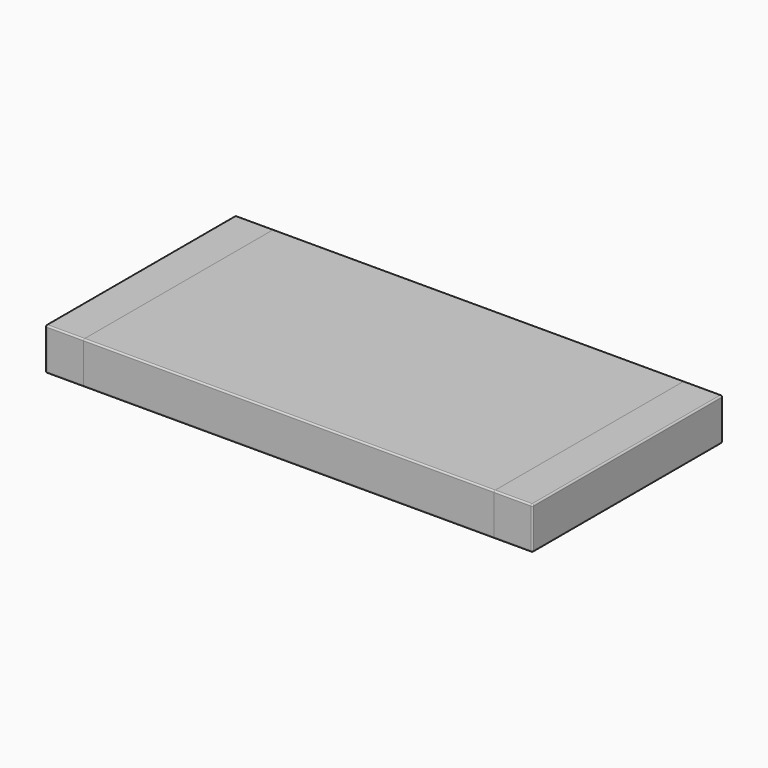
from build123d import *

# Parameters (mm, degrees)
F2_W     = 5.35
F2_H     = 3.1
F3_DEPTH = 0.53
F2_W_2   = 0.5
F4_DEPTH = 0.55
F5_DEPTH = 0.55
F6_DEPTH = 0.02
F7_R     = 0.01999
F7_2_R   = 0.01999
F7_3_R   = 0.01999
F7_4_R   = 0.01999


# Not quite as in the source:
# - a fillet or chamfer is up to 0.001 mm smaller than in the source, because OpenCascade refuses the exact size


with BuildPart() as f3:
    # F2 (on Top) → F3 (new body)
    with BuildSketch(Plane.XY):
        Rectangle(F2_W, F2_H)
    extrude(amount=F3_DEPTH)


with BuildPart() as f4:
    # F2 (on Top) → F4 (new body)
    with BuildSketch(Plane.XY):
        with Locations((-2.925, 0)):
            Rectangle(F2_W_2, F2_H)
    extrude(amount=F4_DEPTH)

    # F7 (radius 0.02 in the source; OpenCascade refuses exactly that, so slightly less here)
    f7_edges = [f4.edges().sort_by_distance(p)[0] for p in [
        (-2.925, -1.55, 0.55),
        (-3.175, 1.55, 0.275),
        (-3.175, -1.55, 0.275),
        (-3.175, 0, 0),
        (-3.175, 0, 0.55),
        (-2.925, 1.55, 0.55),
        (-2.925, 1.55, 0),
        (-2.925, -1.55, 0),
    ]]
    fillet(f7_edges, radius=F7_R)


with BuildPart() as f5:
    # F2 (on Top) → F5 (new body)
    with BuildSketch(Plane.XY):
        with Locations((2.925, 0)):
            Rectangle(F2_W_2, F2_H)
    extrude(amount=F5_DEPTH)

    # F7#2 (radius 0.02 in the source; OpenCascade refuses exactly that, so slightly less here)
    f7_2_edges = [f5.edges().sort_by_distance(p)[0] for p in [
        (2.925, -1.55, 0.55),
        (3.175, -1.55, 0.275),
        (3.175, 1.55, 0.275),
        (3.175, 0, 0),
        (3.175, 0, 0.55),
        (2.925, 1.55, 0.55),
        (2.925, 1.55, 0),
        (2.925, -1.55, 0),
    ]]
    fillet(f7_2_edges, radius=F7_2_R)


with BuildPart() as f6:
    # F6 (new): a face of the model
    f6_faces = [f3.part.faces().sort_by_distance(p)[0] for p in [
        (0, 0, 0.53),
    ]]
    extrude(f6_faces, amount=F6_DEPTH)

    # F7#4 (radius 0.02 in the source; OpenCascade refuses exactly that, so slightly less here)
    f7_4_edges = [f6.edges().sort_by_distance(p)[0] for p in [
        (0, -1.55, 0.55),
        (0, 1.55, 0.55),
    ]]
    fillet(f7_4_edges, radius=F7_4_R)


with BuildPart() as f3_1:
    add(f3.part)

    # F7#3 (radius 0.02 in the source; OpenCascade refuses exactly that, so slightly less here)
    f7_3_edges = [f3_1.edges().sort_by_distance(p)[0] for p in [
        (0, 1.55, 0),
        (0, -1.55, 0),
    ]]
    fillet(f7_3_edges, radius=F7_3_R)


solid = Compound([f4.part, f5.part, f6.part, f3_1.part])
